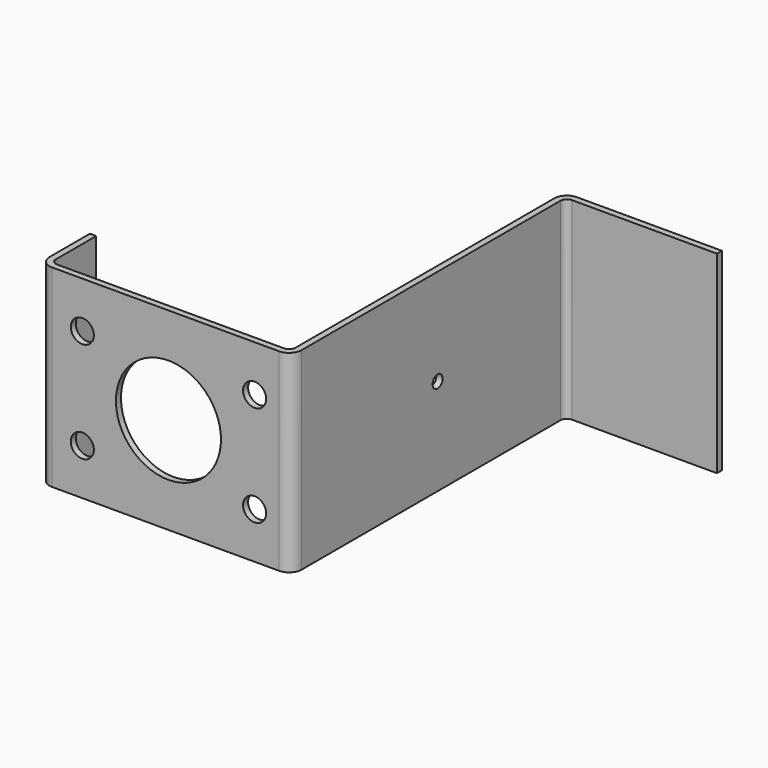
from build123d import *

# Parameters (mm, degrees)
F1_DEPTH = 46
F3_D     = 11
F4_D     = 50
F7_D     = 6


# Not quite as in the source:
# - the program builds the solid bodies; features that only make, move or delete a surface that nothing else refers to are left out


with BuildPart() as f1:
    # F0 (on Top) → F1 (new body, symmetric)
    with BuildSketch(Plane.XY):
        with BuildLine():
            Line((-53.8527505398, 110.754218787), (-53.8527505398, -43.245781213))
            ThreePointArc((-53.8527505398, -43.245781213), (-54.7314301962, -45.3671015566), (-56.8527505398, -46.245781213))
            Line((-56.8527505398, -46.245781213), (-164.8527505398, -46.245781213))
            ThreePointArc((-164.8527505398, -46.245781213), (-166.9740708833, -45.3671015566), (-167.8527505398, -43.245781213))
            Line((-167.8527505398, -43.245781213), (-167.8527505398, -19.245781213))
            Line((-167.8527505398, -19.245781213), (-170.8527505398, -19.245781213))
            Line((-170.8527505398, -19.245781213), (-170.8527505398, -43.245781213))
            ThreePointArc((-170.8527505398, -43.245781213), (-169.0953912269, -47.4884219002), (-164.8527505398, -49.245781213))
            Line((-164.8527505398, -49.245781213), (-56.8527505398, -49.245781213))
            ThreePointArc((-56.8527505398, -49.245781213), (-52.6101098527, -47.4884219002), (-50.8527505398, -43.245781213))
            Line((-50.8527505398, -43.245781213), (-50.8527505398, 110.754218787))
            ThreePointArc((-50.8527505398, 110.754218787), (-49.9740708833, 112.8755391305), (-47.8527505398, 113.754218787))
            Line((-47.8527505398, 113.754218787), (21.1472494602, 113.754218787))
            Line((21.1472494602, 113.754218787), (21.1472494602, 116.754218787))
            Line((21.1472494602, 116.754218787), (-47.8527505398, 116.754218787))
            ThreePointArc((-47.8527505398, 116.754218787), (-52.0953912269, 114.9968594741), (-53.8527505398, 110.754218787))
        make_face()
    extrude(amount=F1_DEPTH, both=True)

    # F3 (through all)
    with Locations(Plane.XZ.offset(49.245781213)):
        with Locations((-150.4841212034, 24), (-68.4841212034, 24), (-68.4841212034, -24), (-150.4841212034, -24)):
            Hole(F3_D / 2)

    # F4 (through all)
    with Locations(Plane.XZ.offset(49.245781213)):
        with Locations((-109.4841212034, 0)):
            Hole(F4_D / 2)

    # F7 (through all)
    with Locations(Plane.YZ.offset(-50.8527505398)):
        with Locations((37.5964443088, 0)):
            Hole(F7_D / 2)


solid = f1.part
